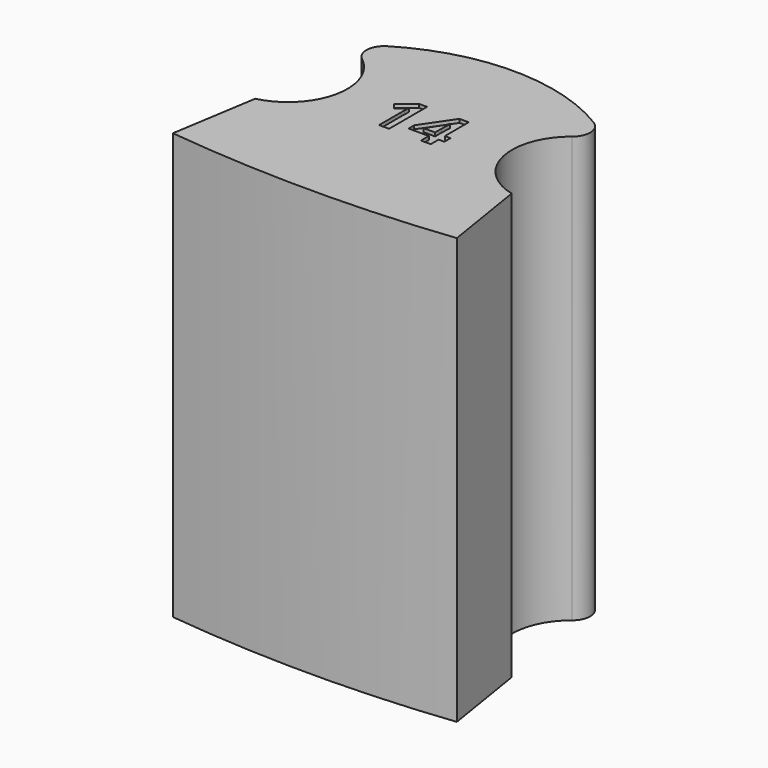
from build123d import *

# Parameters (mm, degrees)
F1_DEPTH     = 120
F2_TEXT_SIZE = 18.7331137972
F3_DEPTH     = 1


# Not quite as in the source:
# - Text() gives the source's letters only with a copy of the font that has no kerning and outlines rounded to 1/6400 em; it was checked with that copy


with BuildPart() as f1:
    # F0 (on Top) → F1 (new body)
    with BuildSketch(Plane.XY):
        with BuildLine():
            Line((3.8687128108, 24.1569802165), (0, 0))
            ThreePointArc((0, 0), (40, -2.2607195109), (80, 0))
            Line((80, 0), (76.1312871892, 24.1569802165))
            ThreePointArc((76.1312871892, 24.1569802165), (63.5975554576, 36.8458138953), (69.5972800683, 53.6417728094))
            ThreePointArc((69.5972800683, 53.6417728094), (71.4969098635, 57.8715436357), (69.1043731597, 61.843359684))
            ThreePointArc((69.1043731597, 61.843359684), (40, 70), (10.8956268403, 61.843359684))
            ThreePointArc((10.8956268403, 61.843359684), (8.5030901365, 57.8715436357), (10.4027199317, 53.6417728094))
            ThreePointArc((10.4027199317, 53.6417728094), (16.4024445424, 36.8458138953), (3.8687128108, 24.1569802165))
        make_face()
    extrude(amount=F1_DEPTH)

    # F2 (on face) → F3 (cut)
    with BuildSketch(Plane.XY.offset(120)):
        with Locations((28.077268973, 31.3721522689)):
            Text('14', F2_TEXT_SIZE, font='Open Sans', font_style=FontStyle.BOLD, text_align=(TextAlign.LEFT, TextAlign.BOTTOM))
    extrude(amount=-F3_DEPTH, mode=Mode.SUBTRACT)


solid = f1.part
